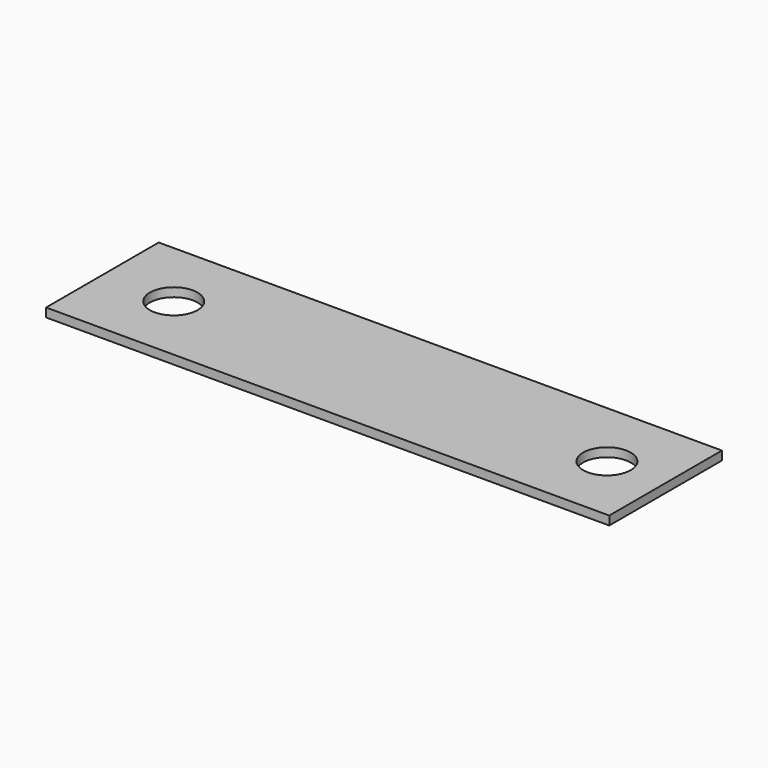
from build123d import *

# Parameters (mm, degrees)
F1_DEPTH = 2.38125


# Not quite as in the source:
# - a feature names something its author has since deleted; it is built from what else it names


with BuildPart() as f1:
    # F0 (on Top) → F1 (new body)
    with BuildSketch(Plane.XY):
        with BuildLine():
            Line((-9.4234, 38.1), (0, 38.1))
            Line((0, 38.1), (0, 57.15))
            Line((0, 57.15), (-152.4, 57.15))
            Line((-152.4, 57.15), (-152.4, 38.1))
            Line((-152.4, 38.1), (-139.5476, 38.1))
            ThreePointArc((-139.5476, 38.1), (-133.096, 44.5516), (-126.6444, 38.1))
            Line((-126.6444, 38.1), (-22.3266, 38.1))
            ThreePointArc((-22.3266, 38.1), (-15.875, 44.5516), (-9.4234, 38.1))
        make_face()
        with BuildLine():
            Line((-152.4, 19.05), (0, 19.05))
            Line((0, 19.05), (0, 38.1))
            Line((0, 38.1), (-9.4234, 38.1))
            ThreePointArc((-9.4234, 38.1), (-15.875, 31.6484), (-22.3266, 38.1))
            Line((-22.3266, 38.1), (-126.6444, 38.1))
            ThreePointArc((-126.6444, 38.1), (-133.096, 31.6484), (-139.5476, 38.1))
            Line((-139.5476, 38.1), (-152.4, 38.1))
            Line((-152.4, 38.1), (-152.4, 19.05))
        make_face()
    extrude(amount=F1_DEPTH)


solid = f1.part
